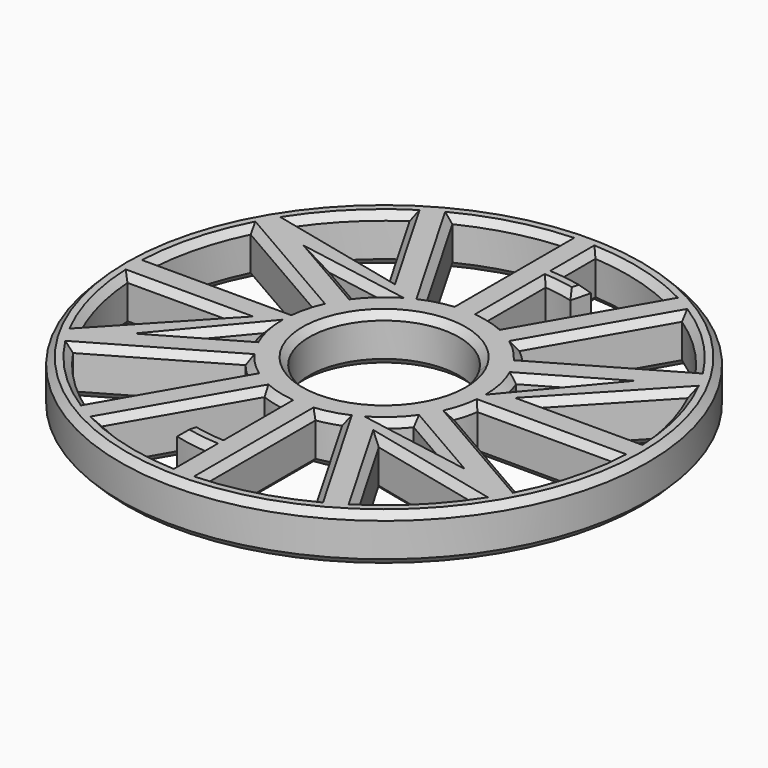
from build123d import *

# Parameters (mm, degrees)
F2_DEPTH           = 7
F3_COUNT           = 12
F5_DEPTH           = 7
F5_COPIES_COUNT    = 2
F5_2_COPIES_COUNT  = 2
F5_2_COPIES_ANGLE  = 120
F5_2_COPIES1_COUNT = 2
F1_R               = 39.1
F6_DEPTH           = 7
F7_DEPTH           = 7
F8_DEPTH           = 25
F9_SIZE            = 1


# Not quite as in the source:
# - a pattern or mirror of a feature is missing from the dataset's text; its kind, count and spacing are read off the source's solid


with BuildPart() as f2:
    # F1 (on Top) → F2 (new body)
    with BuildSketch(Plane.XY):
        with BuildLine():
            Line((2.5, 15.8240908571), (2.5, 36.0133308651))
            ThreePointArc((2.5, 36.0133308651), (0, 36.1), (-2.5, 36.0133308651))
            Line((-2.5, 36.0133308651), (-2.5, 15.8240908571))
            ThreePointArc((-2.5, 15.8240908571), (0, 16.0203574072), (2.5, 15.8240908571))
        make_face()
        with BuildLine():
            ThreePointArc((-2.5, 36.0133308651), (0, 36.1), (2.5, 36.0133308651))
            Line((2.5, 36.0133308651), (2.5, 37.5200061313))
            Line((2.5, 37.5200061313), (-2.5, 37.5200061313))
            Line((-2.5, 37.5200061313), (-2.5, 36.0133308651))
        make_face()
        with BuildLine():
            Line((-2.5, 15.8240908571), (2.5, 15.8240908571))
            ThreePointArc((2.5, 15.8240908571), (0, 16.0203574072), (-2.5, 15.8240908571))
        make_face()
    extrude(amount=F2_DEPTH)


with BuildPart() as f3_1:
    # F3: instance of F2
    add(f2.part.rotate(Axis((0, 0, 0), (0, 0, 1)), 1 * 360 / F3_COUNT))


with BuildPart() as f3_2:
    # F3: instance of F2
    add(f2.part.rotate(Axis((0, 0, 0), (0, 0, 1)), 2 * 360 / F3_COUNT))


with BuildPart() as f3_3:
    # F3: instance of F2
    add(f2.part.rotate(Axis((0, 0, 0), (0, 0, 1)), 3 * 360 / F3_COUNT))


with BuildPart() as f3_4:
    # F3: instance of F2
    add(f2.part.rotate(Axis((0, 0, 0), (0, 0, 1)), 4 * 360 / F3_COUNT))


with BuildPart() as f3_5:
    # F3: instance of F2
    add(f2.part.rotate(Axis((0, 0, 0), (0, 0, 1)), 5 * 360 / F3_COUNT))


with BuildPart() as f3_6:
    # F3: instance of F2
    add(f2.part.rotate(Axis((0, 0, 0), (0, 0, 1)), 6 * 360 / F3_COUNT))


with BuildPart() as f3_7:
    # F3: instance of F2
    add(f2.part.rotate(Axis((0, 0, 0), (0, 0, 1)), 7 * 360 / F3_COUNT))



with BuildPart() as f3_8:
    # F3: instance of F2
    add(f2.part.rotate(Axis((0, 0, 0), (0, 0, 1)), 8 * 360 / F3_COUNT))


with BuildPart() as f3_9:
    # F3: instance of F2
    add(f2.part.rotate(Axis((0, 0, 0), (0, 0, 1)), 9 * 360 / F3_COUNT))



with BuildPart() as f3_10:
    # F3: instance of F2
    add(f2.part.rotate(Axis((0, 0, 0), (0, 0, 1)), 10 * 360 / F3_COUNT))


with BuildPart() as f3_11:
    # F3: instance of F2
    add(f2.part.rotate(Axis((0, 0, 0), (0, 0, 1)), 11 * 360 / F3_COUNT))


with BuildPart() as f2_1:
    add(f2.part)

    # F4 (on Top) → F5 (join)
    with BuildSketch(Plane.XY):
        with BuildLine():
            ThreePointArc((7.4851914007, 28.9646717583), (3.7727157641, 29.677380547), (0, 29.9162213585))
            Line((0, 29.9162213585), (0, 26.9162213585))
            ThreePointArc((0, 26.9162213585), (3.3943876606, 26.7013315142), (6.7345760763, 26.0600931942))
            Line((6.7345760763, 26.0600931942), (7.4851914007, 28.9646717583))
        make_face()
    f5 = extrude(amount=F5_DEPTH)

    # F5_copies: F5 ×2 about axis
    f5_copies_axis = Axis((0, 0, 0), (0, 0, 1))
    for i in range(1, F5_COPIES_COUNT):
        add(f5.rotate(f5_copies_axis, i * 360 / F5_COPIES_COUNT))

    add(f3_1.part)  # F6 merges F3_1

    add(f3_2.part)  # F6 merges F3_2

    add(f3_3.part)  # F6 merges F3_3

    add(f3_4.part)  # F6 merges F3_4

    add(f3_5.part)  # F6 merges F3_5

    add(f3_6.part)  # F6 merges F3_6


with BuildPart() as f3_9_1:
    add(f3_9.part)

    add(f3_10.part)  # F5#2 merges F3_10
    # F4 (on Top) → F5, piece 2 (join)
    with BuildSketch(Plane.XY):
        Polygon((33.7432784599, 16.5949395562), (31.2432784599, 20.9250665751), (15.8240908571, 2.5), (15.8240908571, -2.5), align=None)
    f5_2 = extrude(amount=F5_DEPTH)

    # F5_2_copies: F5#2 ×2 about axis
    f5_2_copies_axis = Axis((0, 0, 0), (0, 0, 1))
    for i in range(1, F5_2_COPIES_COUNT):
        add(f5_2.rotate(f5_2_copies_axis, i * F5_2_COPIES_ANGLE / (F5_2_COPIES_COUNT - 1)))

    # F5_2_copies1: F5#2 ×2 about axis
    f5_2_copies1_axis = Axis((0, 0, 0), (0, 0, 1))
    for i in range(1, F5_2_COPIES1_COUNT):
        add(f5_2.rotate(f5_2_copies1_axis, i * 360 / F5_2_COPIES1_COUNT))


with BuildPart() as f3_7_1:
    add(f3_7.part)

    add(f3_8.part)  # F5#3 merges F3_8
    # F4 (on Top) → F5, piece 3 (join)
    with BuildSketch(Plane.XY):
        Polygon((31.2432784599, -20.9250665751), (33.7432784599, -16.5949395562), (10.077108938, -12.454064674), (5.7469819191, -14.954064674), align=None)
    extrude(amount=F5_DEPTH)


with BuildPart() as f2_2:
    add(f2_1.part)

    add(f3_7_1.part)  # F6 merges F3_7

    add(f3_9_1.part)  # F6 merges F3_9

    add(f3_11.part)  # F6 merges F3_11
    # F1 (on Top) → F6 (join)
    with BuildSketch(Plane.XY):
        Circle(F1_R)
        with BuildLine():
            ThreePointArc((2.5, 36.0133308651), (26.39564358, 24.626814654), (36.1, 0))
            ThreePointArc((36.1, 0), (-24.6268146539, -26.39564358), (-2.5, 36.0133308651))
            Line((-2.5, 36.0133308651), (-2.5, 37.5200061313))
            Line((-2.5, 37.5200061313), (2.5, 37.5200061313))
            Line((2.5, 37.5200061313), (2.5, 36.0133308651))
        make_face(mode=Mode.SUBTRACT)
        with BuildLine():
            ThreePointArc((-2.5, 36.0133308651), (0, 36.1), (2.5, 36.0133308651))
            Line((2.5, 36.0133308651), (2.5, 37.5200061313))
            Line((2.5, 37.5200061313), (-2.5, 37.5200061313))
            Line((-2.5, 37.5200061313), (-2.5, 36.0133308651))
        make_face()
    extrude(amount=F6_DEPTH)

    # F0 (on Top) + F1 (on Top) → F7 (join)
    with BuildSketch(Plane.XY):
        with BuildLine():
            ThreePointArc((9.612881982, 5.55), (10.7217766718, 2.8728914006), (11.1, 0))
            ThreePointArc((11.1, 0), (-2.8728914006, -10.7217766718), (-9.612881982, 5.55))
            Line((-9.612881982, 5.55), (-10.8253175473, 6.25))
            Line((-10.8253175473, 6.25), (-12.2109581934, 7.05))
            ThreePointArc((-12.2109581934, 7.05), (-3.6493485359, -13.6195541507), (14.1, 0))
            ThreePointArc((14.1, 0), (13.6195541507, 3.6493485359), (12.2109581934, 7.05))
            Line((12.2109581934, 7.05), (10.8253175473, 6.25))
            Line((10.8253175473, 6.25), (9.612881982, 5.55))
        make_face()
    with BuildSketch(Plane.XY):
        with BuildLine():
            ThreePointArc((16.0203574072, 0), (12.1799578195, 10.406751605), (2.5, 15.8240908571))
            Line((2.5, 15.8240908571), (-2.5, 15.8240908571))
            ThreePointArc((-2.5, 15.8240908571), (-10.406751605, -12.1799578195), (16.0203574072, 0))
        make_face()
    extrude(amount=F7_DEPTH)

    # F0 (on Top) → F8 (cut)
    with BuildSketch(Plane.XY):
        with BuildLine():
            ThreePointArc((-9.612881982, 5.55), (-2.8728914006, -10.7217766718), (11.1, 0))
            ThreePointArc((11.1, 0), (10.7217766718, 2.8728914006), (9.612881982, 5.55))
            Line((9.612881982, 5.55), (0, 0))
            Line((0, 0), (-9.612881982, 5.55))
        make_face()
        with BuildLine():
            Line((0, 0), (9.612881982, 5.55))
            ThreePointArc((9.612881982, 5.55), (0, 11.1), (-9.612881982, 5.55))
            Line((-9.612881982, 5.55), (0, 0))
        make_face()
    extrude(amount=F8_DEPTH, mode=Mode.SUBTRACT)

    # F9
    f9_edges = [f2_2.edges().sort_by_distance(p)[0] for p in [
        (-39.1, 0, 7),
        (-28.264776, -2.5, 7),
        (-34.929689, -9.117392, 7),
        (-26.578551, -8.960105, 7),
        (-21.196262, -15.124419, 7),
        (-25.526555, -25.526555, 7),
        (-11.328103, -11.328103, 7),
        (-15.124419, -21.196262, 7),
        (-23.696262, 10.794292, 7),
        (-34.869922, 9.343368, 7),
        (-15.474477, 4.146374, 7),
        (-25.918711, 2.5, 7),
        (-18.859494, -6.127136, 7),
        (-18.424481, -7.750627, 7),
        (-15.474477, -4.146374, 7),
        (-11.1, 0, 7),
        (-10.794292, -23.696262, 7),
        (-9.343368, -34.869922, 7),
        (-4.146374, -15.474477, 7),
        (-2.5, -32.912455, 7),
        (-2.5, -21.31198, 7),
        (-5.010521, -29.493643, 7),
        (-4.63208, -26.514653, 7),
        (-7.109884, -27.512382, 7),
        (2.5, -25.918711, 7),
        (9.343368, -34.869922, 7),
        (4.146374, -15.474477, 7),
        (10.794292, -23.696262, 7),
        (21.048954, -18.537648, 7),
        (16.297451, -23.228014, 7),
        (25.360737, -25.691302, 7),
        (14.736003, -13.269232, 7),
        (15.924481, -12.080754, 7),
        (11.328103, -11.328103, 7),
        (-14.736003, 13.269232, 7),
        (-15.924481, 12.080754, 7),
        (-11.328103, 11.328103, 7),
        (-16.297451, 23.228014, 7),
        (-25.360737, 25.691302, 7),
        (-21.048954, 18.537648, 7),
        (-2.5, 25.918711, 7),
        (-9.343368, 34.869922, 7),
        (-4.146374, 15.474477, 7),
        (-10.794292, 23.696262, 7),
        (10.794292, 23.696262, 7),
        (9.343368, 34.869922, 7),
        (4.146374, 15.474477, 7),
        (2.5, 32.912455, 7),
        (2.5, 21.31198, 7),
        (5.010521, 29.493643, 7),
        (4.63208, 26.514653, 7),
        (7.109884, 27.512382, 7),
        (18.859494, 6.127136, 7),
        (18.424481, 7.750627, 7),
        (15.474477, 4.146374, 7),
        (23.696262, -10.794292, 7),
        (34.869922, -9.343368, 7),
        (15.474477, -4.146374, 7),
        (25.918711, -2.5, 7),
        (21.196262, 15.124419, 7),
        (25.526555, 25.526555, 7),
        (11.328103, 11.328103, 7),
        (15.124419, 21.196262, 7),
        (34.929689, 9.117392, 7),
        (26.578551, 8.960105, 7),
        (28.264776, 2.5, 7),
        (-39.1, 0, 0),
        (-28.264776, -2.5, 0),
        (-34.929689, -9.117392, 0),
        (-26.578551, -8.960105, 0),
        (-21.196262, -15.124419, 0),
        (-25.526555, -25.526555, 0),
        (-11.328103, -11.328103, 0),
        (-15.124419, -21.196262, 0),
        (-23.696262, 10.794292, 0),
        (-34.869922, 9.343368, 0),
        (-15.474477, 4.146374, 0),
        (-25.918711, 2.5, 0),
        (-18.859494, -6.127136, 0),
        (-18.424481, -7.750627, 0),
        (-15.474477, -4.146374, 0),
        (-11.1, 0, 0),
        (-10.794292, -23.696262, 0),
        (-9.343368, -34.869922, 0),
        (-4.146374, -15.474477, 0),
        (-2.5, -32.912455, 0),
        (-2.5, -21.31198, 0),
        (-5.010521, -29.493643, 0),
        (-4.63208, -26.514653, 0),
        (-7.109884, -27.512382, 0),
        (2.5, -25.918711, 0),
        (9.343368, -34.869922, 0),
        (4.146374, -15.474477, 0),
        (10.794292, -23.696262, 0),
        (21.048954, -18.537648, 0),
        (16.297451, -23.228014, 0),
        (25.360737, -25.691302, 0),
        (14.736003, -13.269232, 0),
        (15.924481, -12.080754, 0),
        (11.328103, -11.328103, 0),
        (-14.736003, 13.269232, 0),
        (-15.924481, 12.080754, 0),
        (-11.328103, 11.328103, 0),
        (-16.297451, 23.228014, 0),
        (-25.360737, 25.691302, 0),
        (-21.048954, 18.537648, 0),
        (-2.5, 25.918711, 0),
        (-9.343368, 34.869922, 0),
        (-4.146374, 15.474477, 0),
        (-10.794292, 23.696262, 0),
        (10.794292, 23.696262, 0),
        (9.343368, 34.869922, 0),
        (4.146374, 15.474477, 0),
        (2.5, 32.912455, 0),
        (2.5, 21.31198, 0),
        (5.010521, 29.493643, 0),
        (4.63208, 26.514653, 0),
        (7.109884, 27.512382, 0),
        (18.859494, 6.127136, 0),
        (18.424481, 7.750627, 0),
        (15.474477, 4.146374, 0),
        (23.696262, -10.794292, 0),
        (34.869922, -9.343368, 0),
        (15.474477, -4.146374, 0),
        (25.918711, -2.5, 0),
        (21.196262, 15.124419, 0),
        (25.526555, 25.526555, 0),
        (11.328103, 11.328103, 0),
        (15.124419, 21.196262, 0),
        (34.929689, 9.117392, 0),
        (28.264776, 2.5, 0),
        (26.578551, 8.960105, 0),
    ]]
    chamfer(f9_edges, length=F9_SIZE)


solid = f2_2.part
